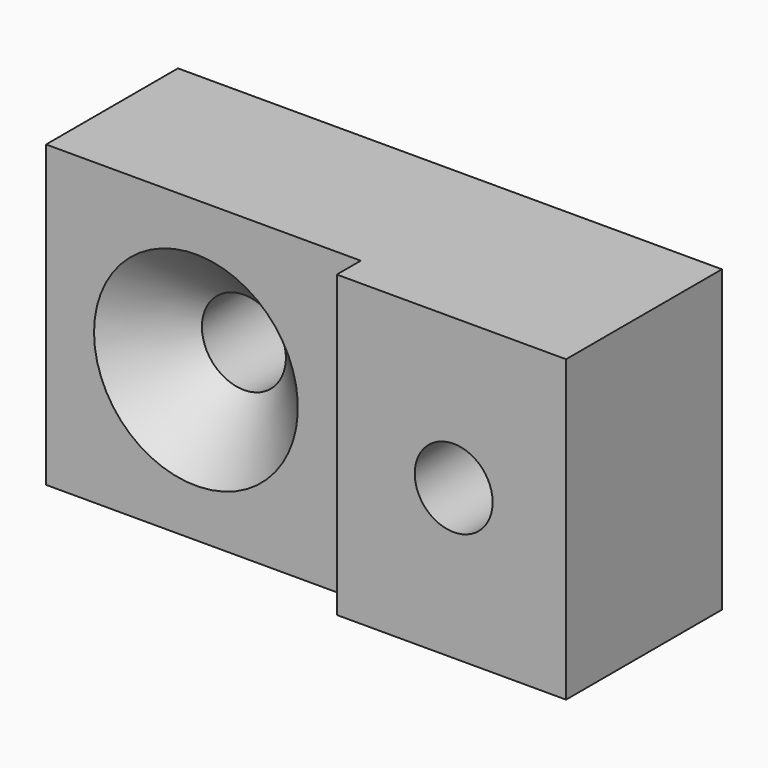
from build123d import *

# Parameters (mm, degrees)
F0_W     = 20
F0_H     = 11
F1_DEPTH = 20
F2_R     = 2.8
F3_DEPTH = 25
F5_DEPTH = 20
F6_R     = 2.6
F7_DEPTH = 25
F8_SIZE  = 4


# Not quite as in the source:
# - a feature names something its author has since deleted; it is built from what else it names


with BuildPart() as f1:
    # F0 (on Top) → F1 (new body)
    with BuildSketch(Plane.XY):
        with Locations((10, 25.5)):
            Rectangle(F0_W, F0_H)
    extrude(amount=F1_DEPTH)

    # F2 (on face) → F3 (cut)
    with BuildSketch(Plane(origin=(0, 31, 0), x_dir=(-1, 0, 0), z_dir=(0, 1, 0))):
        with Locations((-10, 10)):
            Circle(F2_R)
    extrude(amount=-F3_DEPTH, mode=Mode.SUBTRACT)

    # F4 (on face) → F5 (join, through all)
    with BuildSketch(Plane.XY.offset(20)):
        Polygon((21, 20), (21, 18), (36.3, 18), (36.3, 31), (20, 31), (20, 20), align=None)
    extrude(amount=-F5_DEPTH)

    # F6 (on face) → F7 (cut)
    with BuildSketch(Plane.XZ.offset(-18)):
        with Locations((28.8, 10)):
            Circle(F6_R)
    extrude(amount=-F7_DEPTH, mode=Mode.SUBTRACT)

    # F8
    f8_edges = [f1.edges().sort_by_distance(p)[0] for p in [
        (12.8, 20, 10),
    ]]
    chamfer(f8_edges, length=F8_SIZE)


solid = f1.part
